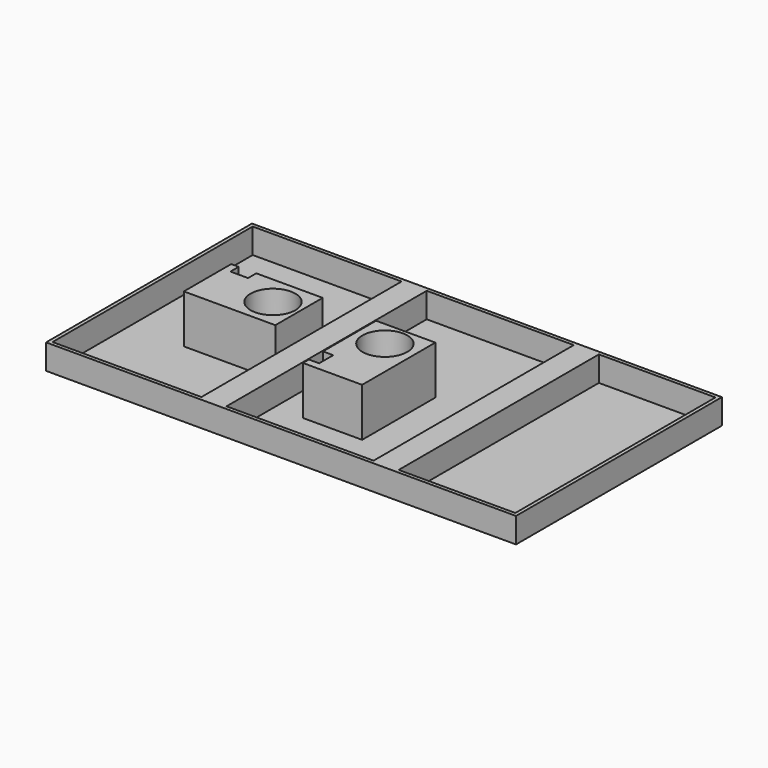
from build123d import *

# Parameters (mm, degrees)
F0_W         = 1663.7
F0_H         = 911.225
F0_W_2       = 88.9
F0_H_2       = 885.825
F1_DEPTH     = 88.9
F2_W         = 1653.4973978996
F2_H         = 894.0463662148
F3_DEPTH     = 1.6256
F4_R         = 79.375
F5_DEPTH     = 171.45
F6_DEPTH     = 1.6266
F7_TEXT_SIZE = 122.4988068624
F8_DEPTH     = 3.175


# Not quite as in the source:
# - Text() gives the source's letters only with a copy of the font that has no kerning and outlines rounded to 1/6400 em; it was checked with that copy


with BuildPart() as f1:
    # F0 (on Top) → F1 (new body)
    with BuildSketch(Plane.XY):
        with Locations((-87.351960619, -263.1033196227)):
            Rectangle(F0_W, F0_H)
        Polygon((-906.501960619, -706.0158196227), (-906.501960619, 179.8091803773), (-379.451960619, 179.8091803773), (-290.551960619, 179.8091803773), (230.148039381, 179.8091803773), (319.048039381, 179.8091803773), (731.798039381, 179.8091803773), (731.798039381, -706.0158196227), (319.048039381, -706.0158196227), (230.148039381, -706.0158196227), (-290.551960619, -706.0158196227), (-379.451960619, -706.0158196227), align=None, mode=Mode.SUBTRACT)
        with Locations((-335.001960619, -263.1033196227)):
            Rectangle(F0_W_2, F0_H_2)
        with Locations((274.598039381, -263.1033196227)):
            Rectangle(F0_W_2, F0_H_2)
    extrude(amount=F1_DEPTH)


with BuildPart() as f3:
    # F2 (on Top) → F3 (new body)
    with BuildSketch(Plane.XY):
        with Locations((-88.077634573, -262.6950442791)):
            Rectangle(F2_W, F2_H)
    extrude(amount=-F3_DEPTH)

    # F4 (on Top) → F6 (cut, through all)
    with BuildSketch(Plane.XY):
        with Locations((-83.8805436191, -263.4980815423)):
            Circle(F4_R)
        with Locations((-481.6117397404, -261.5514993627)):
            Circle(F4_R)
    extrude(amount=-F6_DEPTH, mode=Mode.SUBTRACT)

    # F7 (on face) → F8 (join)
    with BuildSketch(Plane(origin=(0, 0, -1.6256), x_dir=(1, 0, 0), z_dir=(0, 0, -1))):
        with Locations(Location((589.7040041831, 629.8102661108), (0, 0, -90))):
            Text('Shower Head', F7_TEXT_SIZE, font='Open Sans', text_align=(TextAlign.LEFT, TextAlign.BOTTOM))
    extrude(amount=F8_DEPTH)


with BuildPart() as f5:
    # F4 (on Top) → F5 (new body)
    with BuildSketch(Plane.XY):
        Polygon((-713.3867397404, -366.3264993627), (-389.5367397404, -366.3264993627), (-389.5367397404, -156.7764993627), (-624.6218218422, -156.7764993627), (-624.6218218422, -193.1338119316), (-687.0087518311, -193.1338119316), (-687.0087518311, -156.7764993627), (-713.3867397404, -156.7764993627), align=None)
        with Locations((-481.6117397404, -261.5514993627)):
            Circle(F4_R, mode=Mode.SUBTRACT)
    extrude(amount=F5_DEPTH)


with BuildPart() as f5b:
    # F4 (on Top) → F5, piece 2 (new body)
    with BuildSketch(Plane.XY):
        Polygon((20.8944563809, -495.2730815423), (20.8944563809, -171.4230815423), (-188.6555436191, -171.4230815423), (-188.6555436191, -406.5081636441), (-152.2982310502, -406.5081636441), (-152.2982310502, -468.895093633), (-188.6555436191, -468.895093633), (-188.6555436191, -495.2730815423), align=None)
        with Locations((-83.8805436191, -263.4980815423)):
            Circle(F4_R, mode=Mode.SUBTRACT)
    extrude(amount=F5_DEPTH)


solid = Compound([f1.part, f3.part, f5.part, f5b.part])
